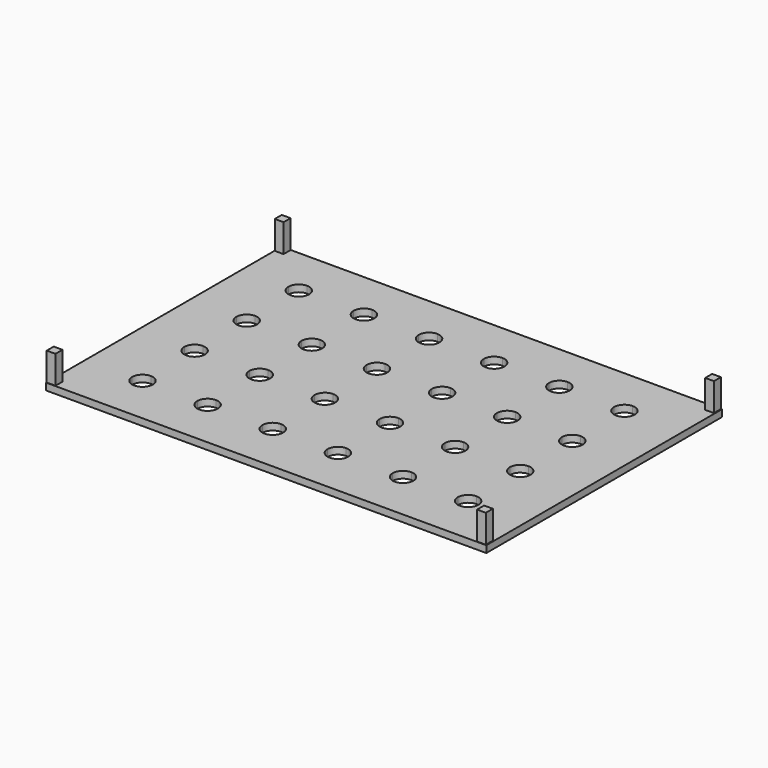
from build123d import *

# Parameters (mm, degrees)
F1_DEPTH = 2
F2_W     = 2.54
F2_H     = 2.54
F3_DEPTH = 10.16


# Not quite as in the source:
# - ends of sketch curves that miss each other by under 0.0002 mm in the source are joined


with BuildPart() as f1:
    # F0 (on Top) → F1 (new body)
    with BuildSketch(Plane.XY):
        with BuildLine():
            Line((-47.4, 31.345), (-47.4, 42.735))
            Line((-47.4, 42.735), (-63.88, 42.735))
            Line((-63.88, 42.735), (-63.88, 28.345))
            Line((-63.88, 28.345), (-50.4, 28.345))
            ThreePointArc((-50.4, 28.345), (-49.52132, 30.46632), (-47.4, 31.345))
        make_face()
        with BuildLine():
            Line((-28.5, 31.345), (-28.5, 42.735))
            Line((-28.5, 42.735), (-47.4, 42.735))
            Line((-47.4, 42.735), (-47.4, 31.345))
            ThreePointArc((-47.4, 31.345), (-45.27868, 30.46632), (-44.4, 28.345))
            Line((-44.4, 28.345), (-31.5, 28.345))
            ThreePointArc((-31.5, 28.345), (-30.62132, 30.46632), (-28.5, 31.345))
        make_face()
        with BuildLine():
            Line((-50.4, 28.345), (-63.88, 28.345))
            Line((-63.88, 28.345), (-63.88, 9.445))
            Line((-63.88, 9.445), (-50.4, 9.445))
            ThreePointArc((-50.4, 9.445), (-49.52132, 11.566321), (-47.4, 12.445))
            Line((-47.4, 12.445), (-47.4, 25.345))
            ThreePointArc((-47.4, 25.345), (-49.52132, 26.22368), (-50.4, 28.345))
        make_face()
        with BuildLine():
            ThreePointArc((-28.5, 25.345), (-30.62132, 26.223679), (-31.5, 28.345))
            Line((-31.5, 28.345), (-44.4, 28.345))
            ThreePointArc((-44.4, 28.345), (-45.27868, 26.22368), (-47.4, 25.345))
            Line((-47.4, 25.345), (-47.4, 12.445))
            ThreePointArc((-47.4, 12.445), (-45.27868, 11.566321), (-44.4, 9.445))
            Line((-44.4, 9.445), (-31.5, 9.445))
            ThreePointArc((-31.5, 9.445), (-30.62132, 11.56632), (-28.5, 12.445))
            Line((-28.5, 12.445), (-28.5, 25.345))
        make_face()
        with BuildLine():
            ThreePointArc((-9.6, 25.345), (-11.721321, 26.223679), (-12.6, 28.345))
            Line((-12.6, 28.345), (-25.5, 28.345))
            ThreePointArc((-25.5, 28.345), (-26.37868, 26.223679), (-28.5, 25.345))
            Line((-28.5, 25.345), (-28.5, 12.445))
            ThreePointArc((-28.5, 12.445), (-26.37868, 11.56632), (-25.5, 9.445))
            Line((-25.5, 9.445), (-12.6, 9.445))
            ThreePointArc((-12.6, 9.445), (-11.721321, 11.566321), (-9.6, 12.445))
            Line((-9.6, 12.445), (-9.6, 25.345))
        make_face()
        with BuildLine():
            Line((-9.6, 31.345), (-9.6, 42.735))
            Line((-9.6, 42.735), (-28.5, 42.735))
            Line((-28.5, 42.735), (-28.5, 31.345))
            ThreePointArc((-28.5, 31.345), (-26.37868, 30.46632), (-25.5, 28.345))
            Line((-25.5, 28.345), (-12.6, 28.345))
            ThreePointArc((-12.6, 28.345), (-11.72132, 30.46632), (-9.6, 31.345))
        make_face()
        with BuildLine():
            ThreePointArc((9.3, 25.345), (7.17868, 26.223679), (6.3, 28.345))
            Line((6.3, 28.345), (-6.6, 28.345))
            ThreePointArc((-6.6, 28.345), (-7.47868, 26.223679), (-9.6, 25.345))
            Line((-9.6, 25.345), (-9.6, 12.445))
            ThreePointArc((-9.6, 12.445), (-7.47868, 11.56632), (-6.6, 9.445))
            Line((-6.6, 9.445), (6.3, 9.445))
            ThreePointArc((6.3, 9.445), (7.17868, 11.56632), (9.3, 12.445))
            Line((9.3, 12.445), (9.3, 25.345))
        make_face()
        with BuildLine():
            Line((9.3, 31.345), (9.3, 42.735))
            Line((9.3, 42.735), (-9.6, 42.735))
            Line((-9.6, 42.735), (-9.6, 31.345))
            ThreePointArc((-9.6, 31.345), (-7.47868, 30.46632), (-6.6, 28.345))
            Line((-6.6, 28.345), (6.3, 28.345))
            ThreePointArc((6.3, 28.345), (7.17868, 30.46632), (9.3, 31.345))
        make_face()
        with BuildLine():
            Line((28.2, 31.345), (28.2, 42.735))
            Line((28.2, 42.735), (9.3, 42.735))
            Line((9.3, 42.735), (9.3, 31.345))
            ThreePointArc((9.3, 31.345), (11.42132, 30.46632), (12.3, 28.345))
            Line((12.3, 28.345), (25.200001, 28.345))
            ThreePointArc((25.200001, 28.345), (26.07868, 30.46632), (28.2, 31.345))
        make_face()
        with BuildLine():
            ThreePointArc((28.2, 25.345), (26.07868, 26.22368), (25.200001, 28.345))
            Line((25.200001, 28.345), (12.3, 28.345))
            ThreePointArc((12.3, 28.345), (11.42132, 26.223679), (9.3, 25.345))
            Line((9.3, 25.345), (9.3, 12.445))
            ThreePointArc((9.3, 12.445), (11.42132, 11.56632), (12.3, 9.445))
            Line((12.3, 9.445), (25.200001, 9.445))
            ThreePointArc((25.200001, 9.445), (26.07868, 11.56632), (28.2, 12.445))
            Line((28.2, 12.445), (28.2, 25.345))
        make_face()
        with BuildLine():
            ThreePointArc((47.1, 25.345), (44.97868, 26.22368), (44.1, 28.345))
            Line((44.1, 28.345), (31.200001, 28.345))
            ThreePointArc((31.200001, 28.345), (30.321321, 26.223679), (28.2, 25.345))
            Line((28.2, 25.345), (28.2, 12.445))
            ThreePointArc((28.2, 12.445), (30.321321, 11.566321), (31.200001, 9.445))
            Line((31.200001, 9.445), (44.1, 9.445))
            ThreePointArc((44.1, 9.445), (44.97868, 11.566321), (47.1, 12.445))
            Line((47.1, 12.445), (47.1, 25.345))
        make_face()
        with BuildLine():
            Line((47.1, 31.345), (47.1, 42.735))
            Line((47.1, 42.735), (28.2, 42.735))
            Line((28.2, 42.735), (28.2, 31.345))
            ThreePointArc((28.2, 31.345), (30.321321, 30.46632), (31.200001, 28.345))
            Line((31.200001, 28.345), (44.1, 28.345))
            ThreePointArc((44.1, 28.345), (44.97868, 30.46632), (47.1, 31.345))
        make_face()
        with BuildLine():
            Line((63.88, 28.345), (63.88, 42.735))
            Line((63.88, 42.735), (47.1, 42.735))
            Line((47.1, 42.735), (47.1, 31.345))
            ThreePointArc((47.1, 31.345), (49.22132, 30.46632), (50.1, 28.345))
            Line((50.1, 28.345), (63.88, 28.345))
        make_face()
        with BuildLine():
            Line((63.88, 9.445), (63.88, 28.345))
            Line((63.88, 28.345), (50.1, 28.345))
            ThreePointArc((50.1, 28.345), (49.22132, 26.22368), (47.1, 25.345))
            Line((47.1, 25.345), (47.1, 12.445))
            ThreePointArc((47.1, 12.445), (49.22132, 11.566321), (50.1, 9.445))
            Line((50.1, 9.445), (63.88, 9.445))
        make_face()
        with BuildLine():
            Line((63.88, -9.455), (63.88, 9.445))
            Line((63.88, 9.445), (50.1, 9.445))
            ThreePointArc((50.1, 9.445), (49.22132, 7.32368), (47.1, 6.445))
            Line((47.1, 6.445), (47.1, -6.455))
            ThreePointArc((47.1, -6.455), (49.22132, -7.33368), (50.1, -9.455))
            Line((50.1, -9.455), (63.88, -9.455))
        make_face()
        with BuildLine():
            Line((47.1, -6.455), (47.1, 6.445))
            ThreePointArc((47.1, 6.445), (44.97868, 7.32368), (44.1, 9.445))
            Line((44.1, 9.445), (31.200001, 9.445))
            ThreePointArc((31.200001, 9.445), (30.321321, 7.32368), (28.2, 6.445))
            Line((28.2, 6.445), (28.2, -6.455))
            ThreePointArc((28.2, -6.455), (30.321321, -7.33368), (31.200001, -9.455))
            Line((31.200001, -9.455), (44.1, -9.455))
            ThreePointArc((44.1, -9.455), (44.97868, -7.33368), (47.1, -6.455))
        make_face()
        with BuildLine():
            ThreePointArc((28.2, 6.445), (26.07868, 7.32368), (25.200001, 9.445))
            Line((25.200001, 9.445), (12.3, 9.445))
            ThreePointArc((12.3, 9.445), (11.42132, 7.32368), (9.3, 6.445))
            Line((9.3, 6.445), (9.3, -6.455))
            ThreePointArc((9.3, -6.455), (11.42132, -7.33368), (12.3, -9.455))
            Line((12.3, -9.455), (25.200001, -9.455))
            ThreePointArc((25.200001, -9.455), (26.07868, -7.33368), (28.2, -6.455))
            Line((28.2, -6.455), (28.2, 6.445))
        make_face()
        with BuildLine():
            ThreePointArc((9.3, 6.445), (7.17868, 7.32368), (6.3, 9.445))
            Line((6.3, 9.445), (-6.6, 9.445))
            ThreePointArc((-6.6, 9.445), (-7.47868, 7.32368), (-9.6, 6.445))
            Line((-9.6, 6.445), (-9.6, -6.455))
            ThreePointArc((-9.6, -6.455), (-7.47868, -7.33368), (-6.6, -9.455))
            Line((-6.6, -9.455), (6.3, -9.455))
            ThreePointArc((6.3, -9.455), (7.17868, -7.33368), (9.3, -6.455))
            Line((9.3, -6.455), (9.3, 6.445))
        make_face()
        with BuildLine():
            ThreePointArc((-9.6, 6.445), (-11.721321, 7.32368), (-12.6, 9.445))
            Line((-12.6, 9.445), (-25.5, 9.445))
            ThreePointArc((-25.5, 9.445), (-26.37868, 7.32368), (-28.5, 6.445))
            Line((-28.5, 6.445), (-28.5, -6.455))
            ThreePointArc((-28.5, -6.455), (-26.37868, -7.33368), (-25.5, -9.455))
            Line((-25.5, -9.455), (-12.6, -9.455))
            ThreePointArc((-12.6, -9.455), (-11.72132, -7.33368), (-9.6, -6.455))
            Line((-9.6, -6.455), (-9.6, 6.445))
        make_face()
        with BuildLine():
            ThreePointArc((-28.5, 6.445), (-30.62132, 7.32368), (-31.5, 9.445))
            Line((-31.5, 9.445), (-44.4, 9.445))
            ThreePointArc((-44.4, 9.445), (-45.27868, 7.32368), (-47.4, 6.445))
            Line((-47.4, 6.445), (-47.4, -6.455))
            ThreePointArc((-47.4, -6.455), (-45.27868, -7.33368), (-44.4, -9.455))
            Line((-44.4, -9.455), (-31.5, -9.455))
            ThreePointArc((-31.5, -9.455), (-30.62132, -7.33368), (-28.5, -6.455))
            Line((-28.5, -6.455), (-28.5, 6.445))
        make_face()
        with BuildLine():
            Line((-50.4, 9.445), (-63.88, 9.445))
            Line((-63.88, 9.445), (-63.88, -9.455))
            Line((-63.88, -9.455), (-50.4, -9.455))
            ThreePointArc((-50.4, -9.455), (-49.52132, -7.33368), (-47.4, -6.455))
            Line((-47.4, -6.455), (-47.4, 6.445))
            ThreePointArc((-47.4, 6.445), (-49.52132, 7.32368), (-50.4, 9.445))
        make_face()
        with BuildLine():
            Line((-50.4, -9.455), (-63.88, -9.455))
            Line((-63.88, -9.455), (-63.88, -28.3526))
            Line((-63.88, -28.3526), (-50.4, -28.3526))
            ThreePointArc((-50.4, -28.3526), (-49.52132, -26.231279), (-47.4, -25.3526))
            Line((-47.4, -25.3526), (-47.4, -12.455))
            ThreePointArc((-47.4, -12.455), (-49.52132, -11.57632), (-50.4, -9.455))
        make_face()
        with BuildLine():
            ThreePointArc((-44.4, -9.455), (-45.27868, -11.57632), (-47.4, -12.455))
            Line((-47.4, -12.455), (-47.4, -25.3526))
            ThreePointArc((-47.4, -25.3526), (-45.27868, -26.231279), (-44.4, -28.3526))
            Line((-44.4, -28.3526), (-31.5, -28.3526))
            ThreePointArc((-31.5, -28.3526), (-30.62132, -26.23128), (-28.5, -25.3526))
            Line((-28.5, -25.3526), (-28.5, -12.455))
            ThreePointArc((-28.5, -12.455), (-30.621321, -11.576321), (-31.5, -9.455))
            Line((-31.5, -9.455), (-44.4, -9.455))
        make_face()
        with BuildLine():
            Line((-25.5, -28.3526), (-12.6, -28.3526))
            ThreePointArc((-12.6, -28.3526), (-11.721321, -26.231279), (-9.6, -25.3526))
            Line((-9.6, -25.3526), (-9.6, -12.455))
            ThreePointArc((-9.6, -12.455), (-11.721321, -11.576321), (-12.6, -9.455))
            Line((-12.6, -9.455), (-25.5, -9.455))
            ThreePointArc((-25.5, -9.455), (-26.37868, -11.576321), (-28.5, -12.455))
            Line((-28.5, -12.455), (-28.5, -25.3526))
            ThreePointArc((-28.5, -25.3526), (-26.37868, -26.23128), (-25.5, -28.3526))
        make_face()
        with BuildLine():
            Line((-6.6, -28.3526), (6.3, -28.3526))
            ThreePointArc((6.3, -28.3526), (7.17868, -26.23128), (9.3, -25.3526))
            Line((9.3, -25.3526), (9.3, -12.455))
            ThreePointArc((9.3, -12.455), (7.17868, -11.576321), (6.3, -9.455))
            Line((6.3, -9.455), (-6.6, -9.455))
            ThreePointArc((-6.6, -9.455), (-7.47868, -11.576321), (-9.6, -12.455))
            Line((-9.6, -12.455), (-9.6, -25.3526))
            ThreePointArc((-9.6, -25.3526), (-7.47868, -26.23128), (-6.6, -28.3526))
        make_face()
        with BuildLine():
            Line((28.2, -25.3526), (28.2, -12.455))
            ThreePointArc((28.2, -12.455), (26.07868, -11.57632), (25.200001, -9.455))
            Line((25.200001, -9.455), (12.3, -9.455))
            ThreePointArc((12.3, -9.455), (11.42132, -11.576321), (9.3, -12.455))
            Line((9.3, -12.455), (9.3, -25.3526))
            ThreePointArc((9.3, -25.3526), (11.42132, -26.23128), (12.3, -28.3526))
            Line((12.3, -28.3526), (25.200001, -28.3526))
            ThreePointArc((25.200001, -28.3526), (26.07868, -26.23128), (28.2, -25.3526))
        make_face()
        with BuildLine():
            Line((47.1, -25.3526), (47.1, -12.455))
            ThreePointArc((47.1, -12.455), (44.97868, -11.57632), (44.1, -9.455))
            Line((44.1, -9.455), (31.200001, -9.455))
            ThreePointArc((31.200001, -9.455), (30.321321, -11.576321), (28.2, -12.455))
            Line((28.2, -12.455), (28.2, -25.3526))
            ThreePointArc((28.2, -25.3526), (30.321321, -26.231279), (31.200001, -28.3526))
            Line((31.200001, -28.3526), (44.1, -28.3526))
            ThreePointArc((44.1, -28.3526), (44.97868, -26.231279), (47.1, -25.3526))
        make_face()
        with BuildLine():
            Line((63.88, -28.3526), (63.88, -9.455))
            Line((63.88, -9.455), (50.1, -9.455))
            ThreePointArc((50.1, -9.455), (49.22132, -11.57632), (47.1, -12.455))
            Line((47.1, -12.455), (47.1, -25.3526))
            ThreePointArc((47.1, -25.3526), (49.22132, -26.231279), (50.1, -28.3526))
            Line((50.1, -28.3526), (63.88, -28.3526))
        make_face()
        with BuildLine():
            Line((63.88, -42.735), (63.88, -28.3526))
            Line((63.88, -28.3526), (50.1, -28.3526))
            ThreePointArc((50.1, -28.3526), (49.22132, -30.47392), (47.1, -31.3526))
            Line((47.1, -31.3526), (47.1, -42.735))
            Line((47.1, -42.735), (63.88, -42.735))
        make_face()
        with BuildLine():
            Line((28.2, -42.735), (47.1, -42.735))
            Line((47.1, -42.735), (47.1, -31.3526))
            ThreePointArc((47.1, -31.3526), (44.97868, -30.47392), (44.1, -28.3526))
            Line((44.1, -28.3526), (31.200001, -28.3526))
            ThreePointArc((31.200001, -28.3526), (30.321321, -30.473921), (28.2, -31.3526))
            Line((28.2, -31.3526), (28.2, -42.735))
        make_face()
        with BuildLine():
            Line((9.3, -42.735), (28.2, -42.735))
            Line((28.2, -42.735), (28.2, -31.3526))
            ThreePointArc((28.2, -31.3526), (26.07868, -30.47392), (25.200001, -28.3526))
            Line((25.200001, -28.3526), (12.3, -28.3526))
            ThreePointArc((12.3, -28.3526), (11.42132, -30.47392), (9.3, -31.3526))
            Line((9.3, -31.3526), (9.3, -42.735))
        make_face()
        with BuildLine():
            Line((-9.6, -42.735), (9.3, -42.735))
            Line((9.3, -42.735), (9.3, -31.3526))
            ThreePointArc((9.3, -31.3526), (7.17868, -30.47392), (6.3, -28.3526))
            Line((6.3, -28.3526), (-6.6, -28.3526))
            ThreePointArc((-6.6, -28.3526), (-7.47868, -30.47392), (-9.6, -31.3526))
            Line((-9.6, -31.3526), (-9.6, -42.735))
        make_face()
        with BuildLine():
            Line((-47.4, -42.735), (-28.5, -42.735))
            Line((-28.5, -42.735), (-28.5, -31.3526))
            ThreePointArc((-28.5, -31.3526), (-30.62132, -30.47392), (-31.5, -28.3526))
            Line((-31.5, -28.3526), (-44.4, -28.3526))
            ThreePointArc((-44.4, -28.3526), (-45.27868, -30.47392), (-47.4, -31.3526))
            Line((-47.4, -31.3526), (-47.4, -42.735))
        make_face()
        with BuildLine():
            Line((-28.5, -42.735), (-9.6, -42.735))
            Line((-9.6, -42.735), (-9.6, -31.3526))
            ThreePointArc((-9.6, -31.3526), (-11.721321, -30.473921), (-12.6, -28.3526))
            Line((-12.6, -28.3526), (-25.5, -28.3526))
            ThreePointArc((-25.5, -28.3526), (-26.37868, -30.47392), (-28.5, -31.3526))
            Line((-28.5, -31.3526), (-28.5, -42.735))
        make_face()
        with BuildLine():
            Line((-50.4, -28.3526), (-63.88, -28.3526))
            Line((-63.88, -28.3526), (-63.88, -42.735))
            Line((-63.88, -42.735), (-47.4, -42.735))
            Line((-47.4, -42.735), (-47.4, -31.3526))
            ThreePointArc((-47.4, -31.3526), (-49.52132, -30.47392), (-50.4, -28.3526))
        make_face()
    extrude(amount=F1_DEPTH)

    # F2 (on Top) → F3 (join)
    with BuildSketch(Plane.XY):
        with Locations((-62.53026, 41.407674)):
            Rectangle(F2_W, F2_H)
        with Locations((-62.53026, -41.325793)):
            Rectangle(F2_W, F2_H)
        with Locations((62.357012, -41.325793)):
            Rectangle(F2_W, F2_H)
        with Locations((62.357012, 41.407674)):
            Rectangle(F2_W, F2_H)
    extrude(amount=F3_DEPTH)


solid = f1.part
